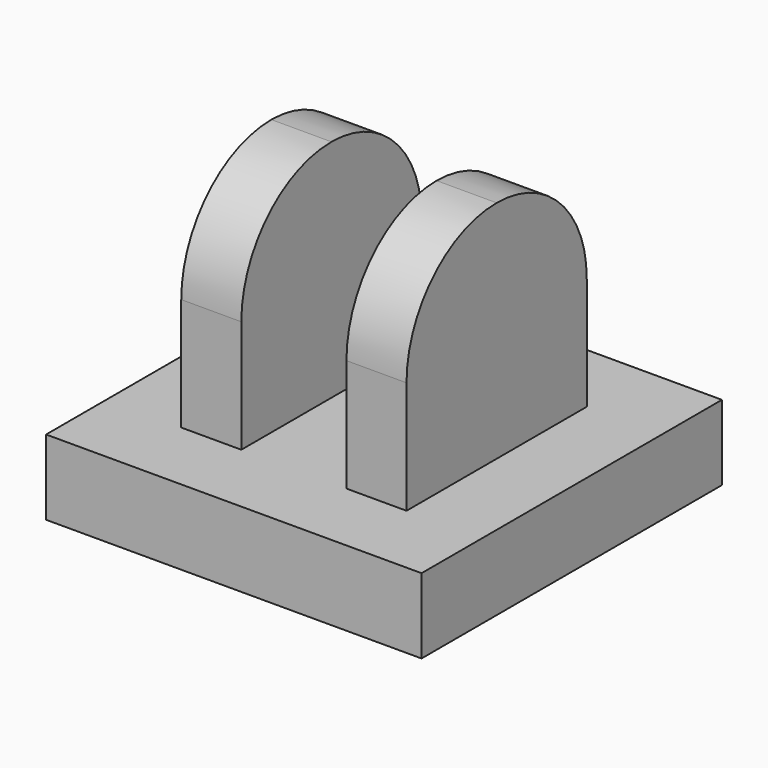
from build123d import *

# Parameters (mm, degrees)
F0_W     = 50
F0_H     = 50
F3_DEPTH = 10
F2_W     = 8
F2_H     = 30
F4_DEPTH = 40
F1_W     = 8
F1_H     = 30
F5_DEPTH = 40
F6_R     = 14.99999
F7_R     = 14.99999


# Not quite as in the source:
# - a fillet or chamfer is up to 0.001 mm smaller than in the source, because OpenCascade refuses the exact size


with BuildPart() as f3:
    # F0 (on Top) → F3 (new body)
    with BuildSketch(Plane.XY):
        with Locations((-0.7709864527, -12.4589413404)):
            Rectangle(F0_W, F0_H)
    extrude(amount=F3_DEPTH)

    # F2 (on face) → F4 (join)
    with BuildSketch(Plane.XY):
        with Locations((10.2290135473, -12.4589413404)):
            Rectangle(F2_W, F2_H)
    extrude(amount=F4_DEPTH)

    # F1 (on face) → F5 (join)
    with BuildSketch(Plane.XY):
        with Locations((-11.7709864527, -12.4589413404)):
            Rectangle(F1_W, F1_H)
    extrude(amount=F5_DEPTH)

    # F6 (radius 15 in the source; OpenCascade refuses exactly that, so slightly less here)
    f6_edges = [f3.edges().sort_by_distance(p)[0] for p in [
        (-11.770986, -27.458941, 40),
        (-11.770986, 2.541059, 40),
    ]]
    fillet(f6_edges, radius=F6_R)

    # F7 (radius 15 in the source; OpenCascade refuses exactly that, so slightly less here)
    f7_edges = [f3.edges().sort_by_distance(p)[0] for p in [
        (10.229014, 2.541059, 40),
        (10.229014, -27.458941, 40),
    ]]
    fillet(f7_edges, radius=F7_R)


solid = f3.part
